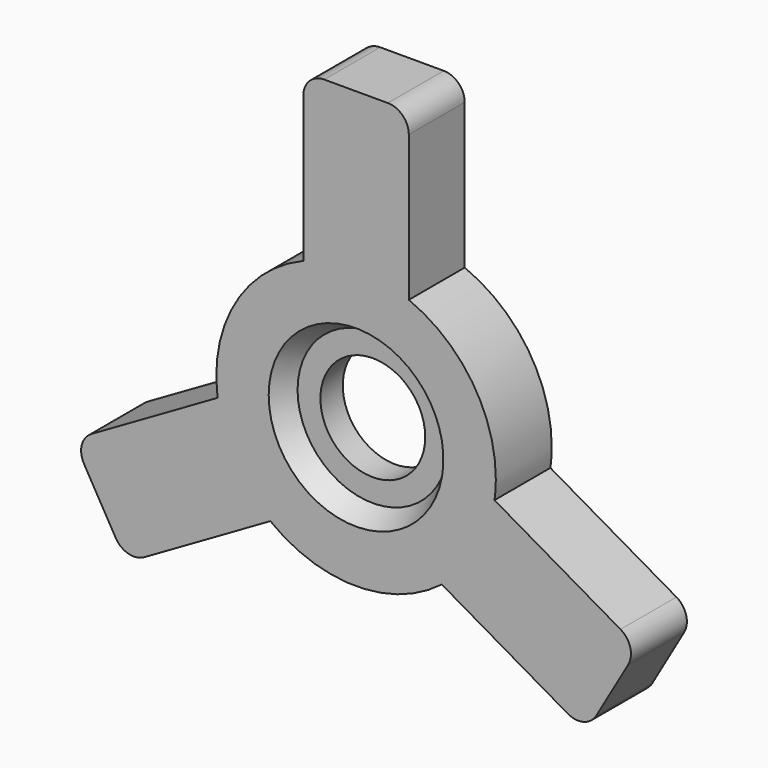
from build123d import *

# Parameters (mm, degrees)
F1_DEPTH = 5
F2_R     = 12.5
F3_DEPTH = 3
F3_TAPER = 30
F4_R     = 7.5
F5_DEPTH = 5.0010001
F6_DEPTH = 5.0010001
F7_R     = 3


# Not quite as in the source:
# - a pattern or mirror of a feature is missing from the dataset's text; its kind, count and spacing are read off the source's solid


with BuildPart() as f1:
    # F0 (on Front) → F1 (new body, symmetric)
    with BuildSketch(Plane.XZ):
        with BuildLine():
            ThreePointArc((19.8138622769, -2.7222897845), (19.9534113066, -1.3643229935), (20, 0))
            ThreePointArc((20, 0), (16.5979995869, 11.1582440246), (7.5493590287, 18.5204529711))
            Line((7.5493590287, 18.5204529711), (-7.5493590287, 18.5204529711))
            ThreePointArc((-7.5493590287, 18.5204529711), (-17.3205080757, 10), (-19.8138622769, -2.7222897845))
            Line((-19.8138622769, -2.7222897845), (-12.2645032483, -15.7981631867))
            ThreePointArc((-12.2645032483, -15.7981631867), (0, -20), (12.2645032483, -15.7981631867))
            Line((12.2645032483, -15.7981631867), (19.8138622769, -2.7222897845))
        make_face()
        with BuildLine():
            Line((-7.5493590287, 18.5204529711), (7.5493590287, 18.5204529711))
            ThreePointArc((7.5493590287, 18.5204529711), (0, 20), (-7.5493590287, 18.5204529711))
        make_face()
        with BuildLine():
            ThreePointArc((-7.5493590287, 18.5204529711), (0, 20), (7.5493590287, 18.5204529711))
            Line((7.5493590287, 18.5204529711), (7.5493590287, 42.3402367583))
            Line((7.5493590287, 42.3402367583), (-7.5493590287, 42.3402367583))
            Line((-7.5493590287, 42.3402367583), (-7.5493590287, 18.5204529711))
        make_face()
        with BuildLine():
            Line((40.4424001493, -14.632181678), (19.8138622769, -2.7222897845))
            ThreePointArc((19.8138622769, -2.7222897845), (17.3205080757, -10), (12.2645032483, -15.7981631867))
            Line((12.2645032483, -15.7981631867), (32.8930411206, -27.7080550803))
            Line((32.8930411206, -27.7080550803), (40.4424001493, -14.632181678))
        make_face()
        with BuildLine():
            ThreePointArc((12.2645032483, -15.7981631867), (17.3205080757, -10), (19.8138622769, -2.7222897845))
            Line((19.8138622769, -2.7222897845), (12.2645032483, -15.7981631867))
        make_face()
        with BuildLine():
            Line((-12.2645032483, -15.7981631867), (-19.8138622769, -2.7222897845))
            ThreePointArc((-19.8138622769, -2.7222897845), (-17.3205080757, -10), (-12.2645032483, -15.7981631867))
        make_face()
        with BuildLine():
            ThreePointArc((-12.2645032483, -15.7981631867), (-17.3205080757, -10), (-19.8138622769, -2.7222897845))
            Line((-19.8138622769, -2.7222897845), (-40.4424001493, -14.632181678))
            Line((-40.4424001493, -14.632181678), (-32.8930411206, -27.7080550803))
            Line((-32.8930411206, -27.7080550803), (-12.2645032483, -15.7981631867))
        make_face()
    extrude(amount=F1_DEPTH, both=True)

    # F2 (on face) → F3 (cut)
    with BuildSketch(Plane(origin=(0, 5, 0), x_dir=(-1, 0, 0), z_dir=(0, 1, 0))):
        Circle(F2_R)
    f3 = extrude(amount=-F3_DEPTH, taper=F3_TAPER, mode=Mode.SUBTRACT)

    # F3_copies: F3 across plane
    add(f3.mirror(Plane(origin=(0, 0, 0), x_dir=(0, 0, -1), z_dir=(0, -1, 0))), mode=Mode.SUBTRACT)

    # F4 (on Front) → F5 (cut, through all)
    with BuildSketch(Plane.XZ):
        Circle(F4_R)
    extrude(amount=-F5_DEPTH, mode=Mode.SUBTRACT)

    # F6 (cut, through all): a face of the model
    f6_faces = [f1.faces().sort_by_distance(p)[0] for p in [
        (0, 0, 0),
    ]]
    extrude(f6_faces, amount=-F6_DEPTH, mode=Mode.SUBTRACT)

    # F7
    f7_edges = [f1.edges().sort_by_distance(p)[0] for p in [
        (-7.549359, 0, 42.340237),
        (7.549359, 0, 42.340237),
        (40.4424, 0, -14.632182),
        (32.893041, 0, -27.708055),
        (-32.893041, 0, -27.708055),
        (-40.4424, 0, -14.632182),
    ]]
    fillet(f7_edges, radius=F7_R)


solid = f1.part
